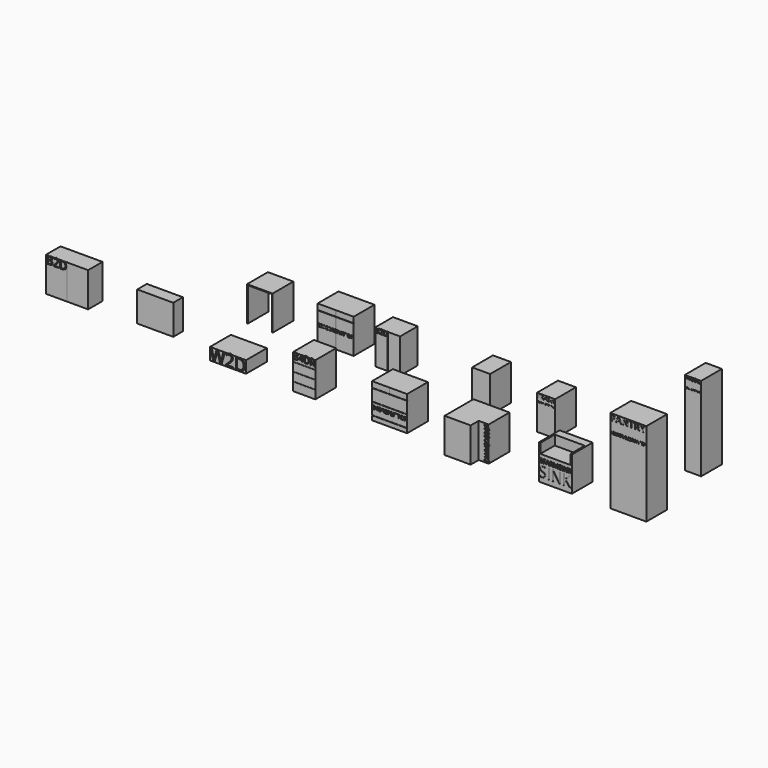
from build123d import *

# Parameters (mm, degrees)
F0_W            = 914.4
F0_H            = 660.4
F1_DEPTH        = 2133.6
F2_TEXT_SIZE    = 225.273693125
F3_DEPTH        = 6.35
F4_W            = 838.2
F4_H            = 660.4
F5_DEPTH        = 876.3
F6_TEXT_SIZE    = 370.8593155894
F7_DEPTH        = 6.35
F9_DEPTH        = 876.3
F10_W           = 889
F10_H           = 660.4
F11_DEPTH       = 876.3
F12_W           = 889
F12_H           = 3.175
F12_H_2         = 6.35
F13_DEPTH       = 12.7
F14_W           = 565.15
F14_H           = 660.4
F15_DEPTH       = 876.3
F16_W           = 914.4
F16_H           = 660.4
F17_DEPTH       = 304.8
F18_W           = 914.4
F18_H           = 304.8
F19_DEPTH       = 762
F20_W           = 1066.8
F20_H           = 457.2
F21_DEPTH       = 876.3
F22_W           = 6.35
F22_H           = 876.3
F23_DEPTH       = 12.7
F24_W           = 457.2
F24_H           = 660.4
F25_DEPTH       = 876.3
F26_TEXT_SIZE   = 149.5033721643
F27_DEPTH       = 6.35
F28_W           = 457.2
F28_H           = 660.4
F29_DEPTH       = 914.4
F30_W           = 628.65
F30_H           = 558.8
F31_DEPTH       = 876.3
F32_W           = 6.35
F32_H           = 876.3
F33_DEPTH       = 6.35
F34_W           = 565.15
F34_H           = 6.35
F35_DEPTH       = 6.35
F36_TEXT_SIZE   = 153.3826073282
F36_TEXT_SIZE_2 = 141.7262423714
F37_DEPTH       = 6.35
F38_W           = 762
F38_H           = 457.2
F39_DEPTH       = 244.475
F40_W           = 412.75
F40_H           = 660.4
F41_DEPTH       = 2133.6
F42_TEXT_SIZE   = 111.7475358518
F43_DEPTH       = 6.35
F44_W           = 914.4
F44_H           = 660.4
F45_DEPTH       = 876.3
F46_W           = 6.35
F46_H           = 876.3
F47_DEPTH       = 6.35
F48_W           = 647.7
F48_H           = 660.4
F49_DEPTH       = 876.3
F50_W           = 609.6
F50_H           = 857.25
F51_DEPTH       = 1153.1221820471
F52_TEXT_SIZE   = 141.7495260963
F53_DEPTH       = 25.4
F54_TEXT_SIZE   = 150.2697554553
F55_DEPTH       = 25.4
F56_TEXT_SIZE   = 43.0312210474
F57_DEPTH       = 25.4
F58_TEXT_SIZE   = 216.1443767181
F59_DEPTH       = 25.4
F60_TEXT_SIZE   = 126.7002182336
F61_DEPTH       = 25.4
F62_TEXT_SIZE   = 108.5855488991
F63_DEPTH       = 25.4
F64_TEXT_SIZE   = 159.3597951344
F65_DEPTH       = 25.4
F66_TEXT_SIZE   = 234.1613316261
F67_DEPTH       = 25.4
F68_TEXT_SIZE   = 271.562099872
F69_DEPTH       = 25.4
F70_TEXT_SIZE   = 97.7069872276
F71_DEPTH       = 25.4
F72_TEXT_SIZE   = 44.1038484014
F73_DEPTH       = 25.4
F74_TEXT_SIZE   = 409.9873896595
F75_DEPTH       = 25.4
F76_W           = 914.5421478271
F76_H           = 12.7
F77_DEPTH       = 12.7
F78_W           = 6.35
F78_H           = 146.05
F79_DEPTH       = 12.7


# Not quite as in the source:
# - Text() gives the source's letters only with a copy of the font that has no kerning and outlines rounded to 1/6400 em; it was checked with that copy


with BuildPart() as f1:
    # F0 (on Top) → F1 (new body)
    with BuildSketch(Plane.XY):
        with Locations((457.2, -330.2)):
            Rectangle(F0_W, F0_H)
    extrude(amount=F1_DEPTH)

    # F2 (on face) → F3 (cut)
    with BuildSketch(Plane.XZ.offset(660.4)):
        with Locations((0, 1971.40294095)):
            Text('PANTRY', F2_TEXT_SIZE, font='Open Sans', font_style=FontStyle.BOLD, text_align=(TextAlign.LEFT, TextAlign.BOTTOM))
    extrude(amount=-F3_DEPTH, mode=Mode.SUBTRACT)

    # F70 (on face) → F71 (cut)
    with BuildSketch(Plane.XZ.offset(660.4)):
        with Locations((0, 1670.7873963279)):
            Text('LOWER-T2DPANTRY', F70_TEXT_SIZE, font='Open Sans', text_align=(TextAlign.LEFT, TextAlign.BOTTOM))
    extrude(amount=-F71_DEPTH, mode=Mode.SUBTRACT)


with BuildPart() as f5:
    # F4 (on Top) → F5 (new body)
    with BuildSketch(Plane.XY):
        with Locations((-1405.5967244318, -317.2923885286)):
            Rectangle(F4_W, F4_H)
    extrude(amount=F5_DEPTH)

    # F6 (on face) → F7 (cut)
    with BuildSketch(Plane.XZ.offset(647.4923885286)):
        with Locations((-1824.6967244318, 121.9596316313)):
            Text('SINK', F6_TEXT_SIZE, font='Open Sans', text_align=(TextAlign.LEFT, TextAlign.BOTTOM))
    extrude(amount=-F7_DEPTH, mode=Mode.SUBTRACT)

    # F38 (on face) → F39 (cut)
    with BuildSketch(Plane.XY.offset(876.3)):
        with Locations((-1405.5967244318, -418.8923885286)):
            Rectangle(F38_W, F38_H)
    extrude(amount=-F39_DEPTH, mode=Mode.SUBTRACT)

    # F54 (on face) → F55 (cut)
    with BuildSketch(Plane.XZ.offset(647.4923885286)):
        with Locations((-1824.6967244318, 438.15)):
            Text('BFARMSINK', F54_TEXT_SIZE, font='Open Sans', text_align=(TextAlign.LEFT, TextAlign.BOTTOM))
    extrude(amount=-F55_DEPTH, mode=Mode.SUBTRACT)


with BuildPart() as f9:
    # F8 (on Top) → F9 (new body)
    with BuildSketch(Plane.XY):
        Polygon((-3079.833200264, -9.8356608667), (-3994.233200264, -9.8356608667), (-3994.233200264, -924.2356608667), (-3333.833200264, -924.2356608667), (-3333.833200264, -670.2356608667), (-3079.833200264, -670.2356608667), align=None)
    extrude(amount=F9_DEPTH)

    # F52 (on face) → F53 (cut)
    with BuildSketch(Plane.XZ.offset(670.2356608667)):
        with Locations(Location((-3181.8928590533, 876.3), (0, 0, -90))):
            Text('B90SUSANV2', F52_TEXT_SIZE, font='Open Sans', text_align=(TextAlign.LEFT, TextAlign.BOTTOM))
    extrude(amount=-F53_DEPTH, mode=Mode.SUBTRACT)


with BuildPart() as f11:
    # F10 (on Top) → F11 (new body)
    with BuildSketch(Plane.XY):
        with Locations((-5602.2624664307, -330.2)):
            Rectangle(F10_W, F10_H)
    extrude(amount=F11_DEPTH)

    # F12 (on face) → F13 (cut)
    with BuildSketch(Plane.XZ.offset(660.4)):
        with Locations((-5602.2624664307, 728.6625)):
            Rectangle(F12_W, F12_H)
        with Locations((-5602.2624664307, 725.4875)):
            Rectangle(F12_W, F12_H)
        with Locations((-5602.2624664307, 422.275)):
            Rectangle(F12_W, F12_H)
        with Locations((-5602.2624664307, 419.1)):
            Rectangle(F12_W, F12_H)
        with Locations((-5602.2624664307, 114.3)):
            Rectangle(F12_W, F12_H_2)
    extrude(amount=-F13_DEPTH, mode=Mode.SUBTRACT)

    # F60 (on face) → F61 (cut)
    with BuildSketch(Plane.XZ.offset(660.4)):
        with Locations((-6046.7624664307, 260.6617830483)):
            Text('B4DRSPLITTOP', F60_TEXT_SIZE, font='Open Sans', text_align=(TextAlign.LEFT, TextAlign.BOTTOM))
    extrude(amount=-F61_DEPTH, mode=Mode.SUBTRACT)

    # F78 (on face) → F79 (cut)
    with BuildSketch(Plane.XZ.offset(660.4)):
        with Locations((-5602.2624664307, 803.275)):
            Rectangle(F78_W, F78_H)
    extrude(amount=-F79_DEPTH, mode=Mode.SUBTRACT)


with BuildPart() as f15:
    # F14 (on Top) → F15 (new body)
    with BuildSketch(Plane.XY):
        with Locations((-7768.1710023851, -330.2)):
            Rectangle(F14_W, F14_H)
    extrude(amount=F15_DEPTH)

    # F34 (on face) → F35 (cut)
    with BuildSketch(Plane.XZ.offset(660.4)):
        with Locations((-7768.1710023851, 658.8125)):
            Rectangle(F34_W, F34_H)
        with Locations((-7768.1710023851, 438.15)):
            Rectangle(F34_W, F34_H)
        with Locations((-7768.1710023851, 217.4875)):
            Rectangle(F34_W, F34_H)
    extrude(amount=-F35_DEPTH, mode=Mode.SUBTRACT)

    # F58 (on face) → F59 (cut)
    with BuildSketch(Plane.XZ.offset(660.4)):
        with Locations((-8050.7460023851, 722.2032816276)):
            Text('B4DR', F58_TEXT_SIZE, font='Open Sans', text_align=(TextAlign.LEFT, TextAlign.BOTTOM))
    extrude(amount=-F59_DEPTH, mode=Mode.SUBTRACT)


with BuildPart() as f17:
    # F16 (on Top) → F17 (new body)
    with BuildSketch(Plane.XY):
        with Locations((-9701.7107513428, -330.2)):
            Rectangle(F16_W, F16_H)
    extrude(amount=F17_DEPTH)

    # F74 (on face) → F75 (cut)
    with BuildSketch(Plane.XZ.offset(660.4)):
        with Locations((-10158.9107513428, 9.6090794451)):
            Text('W2D', F74_TEXT_SIZE, font='Open Sans', text_align=(TextAlign.LEFT, TextAlign.BOTTOM))
    extrude(amount=-F75_DEPTH, mode=Mode.SUBTRACT)


with BuildPart() as f19:
    # F18 (on Top) → F19 (new body)
    with BuildSketch(Plane.XY):
        with Locations((-11819.0208633145, -171.0750684142)):
            Rectangle(F18_W, F18_H)
    extrude(amount=F19_DEPTH)


with BuildPart() as f21:
    # F20 (on Top) → F21 (new body)
    with BuildSketch(Plane.XY):
        with Locations((-13948.7434020996, -228.6)):
            Rectangle(F20_W, F20_H)
    extrude(amount=F21_DEPTH)

    # F22 (on face) → F23 (cut)
    with BuildSketch(Plane.XZ.offset(457.2)):
        with Locations((-13948.7434020996, 438.15)):
            Rectangle(F22_W, F22_H)
    extrude(amount=-F23_DEPTH, mode=Mode.SUBTRACT)

    # F68 (on face) → F69 (cut)
    with BuildSketch(Plane.XZ.offset(457.2)):
        with Locations((-14482.1434020996, 680.7752880922)):
            Text('B2D', F68_TEXT_SIZE, font='Open Sans', text_align=(TextAlign.LEFT, TextAlign.BOTTOM))
    extrude(amount=-F69_DEPTH, mode=Mode.SUBTRACT)


with BuildPart() as f25:
    # F24 (on Top) → F25 (new body)
    with BuildSketch(Plane.XY):
        with Locations((-2956.4073085785, 1327.9767761581)):
            Rectangle(F24_W, F24_H)
    extrude(amount=F25_DEPTH)

    # F26 (on face) → F27 (cut)
    with BuildSketch(Plane.XZ.offset(-997.7767761581)):
        with Locations((-3185.0073085785, 768.6575720417)):
            Text('TRASH', F26_TEXT_SIZE, font='Open Sans', text_align=(TextAlign.LEFT, TextAlign.BOTTOM))
    extrude(amount=-F27_DEPTH, mode=Mode.SUBTRACT)

    # F56 (on face) → F57 (cut)
    with BuildSketch(Plane.XZ.offset(-997.7767761581)):
        with Locations((-3185.0073085785, 671.3806044065)):
            Text('B1DR1PULLOUTTRASH', F56_TEXT_SIZE, font='Open Sans', text_align=(TextAlign.LEFT, TextAlign.BOTTOM))
    extrude(amount=-F57_DEPTH, mode=Mode.SUBTRACT)


with BuildPart() as f29:
    # F28 (on Top) → F29 (new body)
    with BuildSketch(Plane.XY):
        with Locations((-4593.0812358856, 1312.3372465617)):
            Rectangle(F28_W, F28_H)
    extrude(amount=F29_DEPTH)

    # F36 (on face) → F37 (cut)
    with BuildSketch(Plane(origin=(0, 1642.5372465617, 0), x_dir=(-1, 0, 0), z_dir=(0, 1, 0))):
        with Locations((-4821.6812358856, 803.9645227237)):
            Text('MIXER', F36_TEXT_SIZE, font='Open Sans', text_align=(TextAlign.LEFT, TextAlign.BOTTOM))
        with Locations((4364.4812358856, 812.3571054926)):
            Text('MIXER', F36_TEXT_SIZE_2, font='Open Sans', font_style=FontStyle.BOLD, text_align=(TextAlign.LEFT, TextAlign.BOTTOM))
    extrude(amount=-F37_DEPTH, mode=Mode.SUBTRACT)

    # F66 (on face) → F67 (cut)
    with BuildSketch(Plane(origin=(0, 1642.5372465617, 0), x_dir=(-1, 0, 0), z_dir=(0, 1, 0))):
        with Locations((4364.4812358856, 495.8881304171)):
            Text('B1D', F66_TEXT_SIZE, font='Open Sans', text_align=(TextAlign.LEFT, TextAlign.BOTTOM))
    extrude(amount=-F67_DEPTH, mode=Mode.SUBTRACT)


with BuildPart() as f31:
    # F30 (on Top) → F31 (new body)
    with BuildSketch(Plane.XY):
        with Locations((-7125.7337272819, 1464.3686711788)):
            Rectangle(F30_W, F30_H)
    extrude(amount=F31_DEPTH)

    # F32 (on face) → F33 (cut)
    with BuildSketch(Plane.XZ.offset(-1184.9686711788)):
        with Locations((-7125.7337272819, 438.15)):
            Rectangle(F32_W, F32_H)
    extrude(amount=-F33_DEPTH, mode=Mode.SUBTRACT)

    # F64 (on face) → F65 (cut)
    with BuildSketch(Plane.XZ.offset(-1184.9686711788)):
        with Locations((-7440.0587272819, 761.5609475032)):
            Text('B2D', F64_TEXT_SIZE, font='Open Sans', text_align=(TextAlign.LEFT, TextAlign.BOTTOM))
    extrude(amount=-F65_DEPTH, mode=Mode.SUBTRACT)


with BuildPart() as f41:
    # F40 (on Top) → F41 (new body)
    with BuildSketch(Plane.XY):
        with Locations((340.7268749744, 1865.2507066727)):
            Rectangle(F40_W, F40_H)
    extrude(amount=F41_DEPTH)

    # F42 (on face) → F43 (cut)
    with BuildSketch(Plane.XZ.offset(-1535.0507066727)):
        with Locations((134.3518749744, 2053.1417741867)):
            Text('BROOM', F42_TEXT_SIZE, font='Open Sans', text_align=(TextAlign.LEFT, TextAlign.BOTTOM))
    extrude(amount=-F43_DEPTH, mode=Mode.SUBTRACT)

    # F72 (on face) → F73 (cut)
    with BuildSketch(Plane.XZ.offset(-1535.0507066727)):
        with Locations((134.3518749744, 1846.1468885429)):
            Text('LOWER-T1DPANTRY', F72_TEXT_SIZE, font='Open Sans', text_align=(TextAlign.LEFT, TextAlign.BOTTOM))
    extrude(amount=-F73_DEPTH, mode=Mode.SUBTRACT)


with BuildPart() as f45:
    # F44 (on Top) → F45 (new body)
    with BuildSketch(Plane.XY):
        with Locations((-8514.8935317993, 1599.5698650075)):
            Rectangle(F44_W, F44_H)
    extrude(amount=F45_DEPTH)

    # F46 (on face) → F47 (cut)
    with BuildSketch(Plane.XZ.offset(-1269.3698650075)):
        with Locations((-8514.8935317993, 438.15)):
            Rectangle(F46_W, F46_H)
    extrude(amount=-F47_DEPTH, mode=Mode.SUBTRACT)

    # F62 (on face) → F63 (cut)
    with BuildSketch(Plane.XZ.offset(-1269.3698650075)):
        with Locations((-8972.0935317993, 367.5052234012)):
            Text('B2D2DRSPLITTOP', F62_TEXT_SIZE, font='Open Sans', text_align=(TextAlign.LEFT, TextAlign.BOTTOM))
    extrude(amount=-F63_DEPTH, mode=Mode.SUBTRACT)

    # F76 (on face) → F77 (cut)
    with BuildSketch(Plane.XZ.offset(-1269.3698650075)):
        with Locations((-8514.9646057129, 729.5702887535)):
            Rectangle(F76_W, F76_H)
    extrude(amount=-F77_DEPTH, mode=Mode.SUBTRACT)


with BuildPart() as f49:
    # F48 (on Top) → F49 (new body)
    with BuildSketch(Plane.XY):
        with Locations((-10257.8234672546, 1372.5295247256)):
            Rectangle(F48_W, F48_H)
    extrude(amount=F49_DEPTH)

    # F50 (on face) → F51 (cut, through all)
    with BuildSketch(Plane.XZ.offset(-1042.3295247256)):
        with Locations((-10257.8234672546, 428.625)):
            Rectangle(F50_W, F50_H)
    extrude(amount=-F51_DEPTH, mode=Mode.SUBTRACT)


solid = Compound([f1.part, f5.part, f9.part, f11.part, f15.part, f17.part, f19.part, f21.part, f25.part, f29.part, f31.part, f41.part, f45.part, f49.part])
